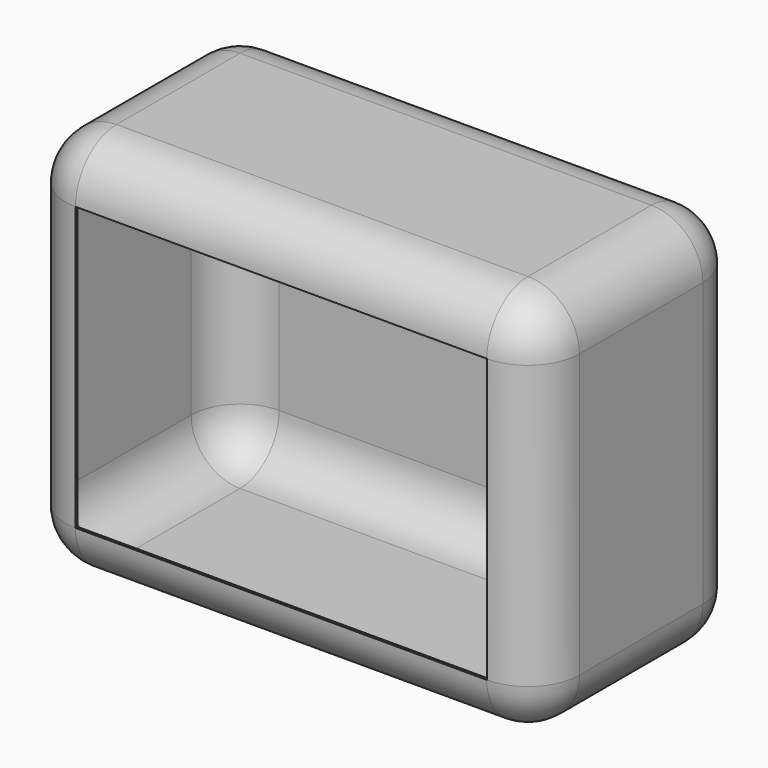
from build123d import *

# Parameters (mm, degrees)
F0_W     = 50.8
F0_H     = 38.1
F1_DEPTH = 25.4
F2_R     = 5.08
F3_T     = -0.254


# Not quite as in the source:
# - a shell that OpenCascade refuses in one call is made with other operations: the cavity is built on its own and cut out


with BuildPart() as f1:
    # F0 (on Front) → F1 (new body)
    with BuildSketch(Plane.XZ):
        with Locations((25.4, 19.05)):
            Rectangle(F0_W, F0_H)
    extrude(amount=F1_DEPTH)

    # F2
    f2_edges = [f1.edges().sort_by_distance(p)[0] for p in [
        (50.8, -12.7, 38.1),
        (25.4, -25.4, 38.1),
        (25.4, 0, 38.1),
        (50.8, -25.4, 19.05),
        (50.8, 0, 19.05),
        (50.8, -12.7, 0),
        (25.4, -25.4, 0),
        (25.4, 0, 0),
        (0, -25.4, 19.05),
        (0, -12.7, 38.1),
        (0, -12.7, 0),
        (0, 0, 19.05),
    ]]
    fillet(f2_edges, radius=F2_R)

    # F3: a shell. OpenCascade refuses it in one call, so the cavity is built on its own and cut out:
    # the body offset inwards by the wall thickness, plus a prism from it out through each open face.
    f3_core = offset(f1.part, amount=F3_T, mode=Mode.PRIVATE)
    f3_exits = [f3_core.faces().sort_by_distance(p)[0] for p in [
        (25.4, -25.146, 19.05),
    ]]
    add(f3_core, mode=Mode.SUBTRACT)
    extrude(f3_exits, amount=-F3_T, mode=Mode.SUBTRACT)


solid = f1.part
